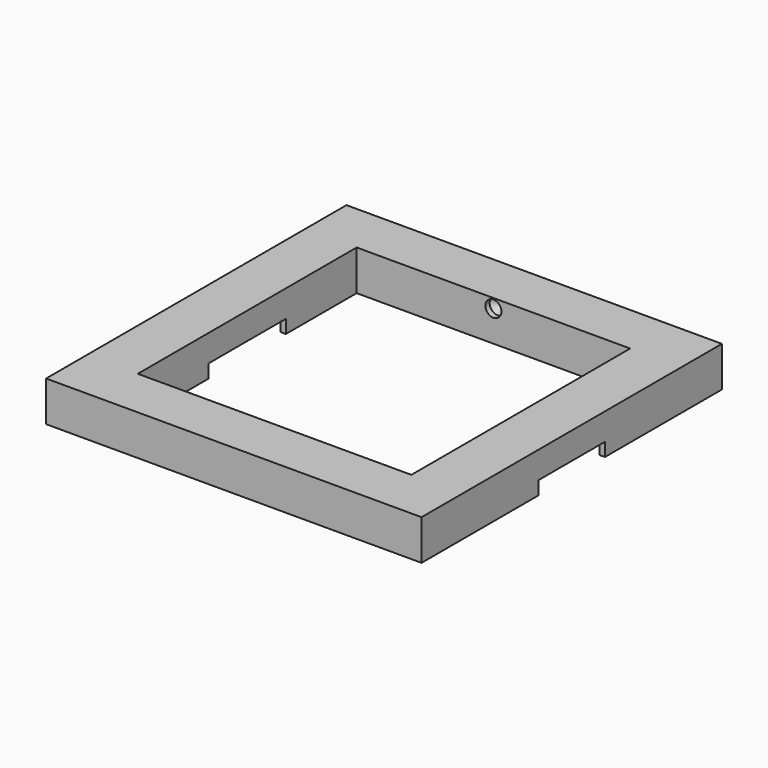
from build123d import *

# Parameters (mm, degrees)
F1_DEPTH = 10
F2_DEPTH = 5
F3_D     = 2
F3_DEPTH = 4
F3_TIP   = 0.600860619
F4_R     = 5
F6_D     = 6
F6_DEPTH = 2
F6_TIP   = 1.8025818571
F8_D     = 6
F8_DEPTH = 2
F8_TIP   = 1.8025818571


# Not quite as in the source:
# - a feature names something its author has since deleted; it is built from what else it names


with BuildPart() as f1:
    # F0 (on Top) → F1 (new body)
    with BuildSketch(Plane.XY):
        Polygon((70, 70), (-70, 70), (-70, 15.5), (-68, 15.5), (-68, 68), (68, 68), (68, 15.5), (70, 15.5), align=None)
        Polygon((-68, 68), (-68, 15.5), (-68, 0), (-68, -15.5), (-68, -68), (68, -68), (68, -15.5), (68, 0), (68, 15.5), (68, 68), align=None)
        Polygon((53, -18), (53, -53), (-53, -53), (-53, -18), (-53, 18), (-53, 53), (53, 53), (53, 18), (53, 0), align=None, mode=Mode.SUBTRACT)
        Polygon((-68, 15.5), (-70, 15.5), (-70, -15.5), (-68, -15.5), (-68, 0), align=None)
        Polygon((-68, -15.5), (-70, -15.5), (-70, -70), (70, -70), (70, -15.5), (68, -15.5), (68, -68), (-68, -68), align=None)
        Polygon((70, -15.5), (70, 15.5), (68, 15.5), (68, 0), (68, -15.5), align=None)
        Polygon((-53, 53), (-53, 18), (-51, 18), (-51, 51), (51, 51), (51, 18), (53, 18), (53, 53), align=None)
        Polygon((-53, 18), (-53, -18), (-51, -18), (-51, 0), (-51, 18), align=None)
        Polygon((51, -18), (53, -18), (53, 0), (53, 18), (51, 18), align=None)
        Polygon((-53, -53), (53, -53), (53, -18), (51, -18), (51, -51), (-51, -51), (-51, -18), (-53, -18), align=None)
    extrude(amount=F1_DEPTH)

    # F0 (on Top) → F2 (join)
    with BuildSketch(Plane.XY):
        Polygon((70, 70), (-70, 70), (-70, 15.5), (-68, 15.5), (-68, 68), (68, 68), (68, 15.5), (70, 15.5), align=None)
        Polygon((-68, -15.5), (-70, -15.5), (-70, -70), (70, -70), (70, -15.5), (68, -15.5), (68, -68), (-68, -68), align=None)
        Polygon((-53, -53), (53, -53), (53, -18), (51, -18), (51, -51), (-51, -51), (-51, -18), (-53, -18), align=None)
        Polygon((-53, 53), (-53, 18), (-51, 18), (-51, 51), (51, 51), (51, 18), (53, 18), (53, 53), align=None)
    extrude(amount=-F2_DEPTH)

    # F3
    with Locations(Plane(origin=(0, 0, 0), x_dir=(1, 0, 0), z_dir=(0, 0, -1))):
        with Locations((0, 60.5), (60.5, 0), (0, -60.5), (-60.5, 0), (-60.5, 40), (-40, 60.5), (40, 60.5), (60.5, 40), (60.5, -40), (40, -60.5), (-40, -60.5), (-60.5, -40)):
            Hole(F3_D / 2, depth=F3_DEPTH)
            with Locations((0, 0, -(F3_DEPTH + F3_TIP / 2))):  # 118° drill point
                Cone(0, F3_D / 2, F3_TIP, mode=Mode.SUBTRACT)

    # F4
    f4_edges = [f1.edges().sort_by_distance(p)[0] for p in [
        (-68, -68, -2.5),
        (-53, -53, -2.5),
        (-53, 53, -2.5),
        (53, 53, -2.5),
        (53, -53, -2.5),
        (68, 68, -2.5),
        (-68, 68, -2.5),
        (68, -68, -2.5),
    ]]
    fillet(f4_edges, radius=F4_R)

    # F6 (one way)
    with BuildSketch(Plane.XZ.offset(-51)):
        with Locations((0, 6.5)):
            Circle(F6_D / 2)
    extrude(amount=-F6_DEPTH, mode=Mode.SUBTRACT)
    with Locations(Plane.XZ.offset(-51)):
        with Locations((0, 6.5)):
            with Locations((0, 0, -(F6_DEPTH + F6_TIP / 2))):  # 118° drill point
                Cone(0, F6_D / 2, F6_TIP, mode=Mode.SUBTRACT)

    # F8 (one way)
    with BuildSketch(Plane(origin=(0, -51, 0), x_dir=(-1, 0, 0), z_dir=(0, 1, 0))):
        with Locations((0, 6.5)):
            Circle(F8_D / 2)
    extrude(amount=-F8_DEPTH, mode=Mode.SUBTRACT)
    with Locations(Plane(origin=(0, -51, 0), x_dir=(-1, 0, 0), z_dir=(0, 1, 0))):
        with Locations((0, 6.5)):
            with Locations((0, 0, -(F8_DEPTH + F8_TIP / 2))):  # 118° drill point
                Cone(0, F8_D / 2, F8_TIP, mode=Mode.SUBTRACT)


solid = f1.part
